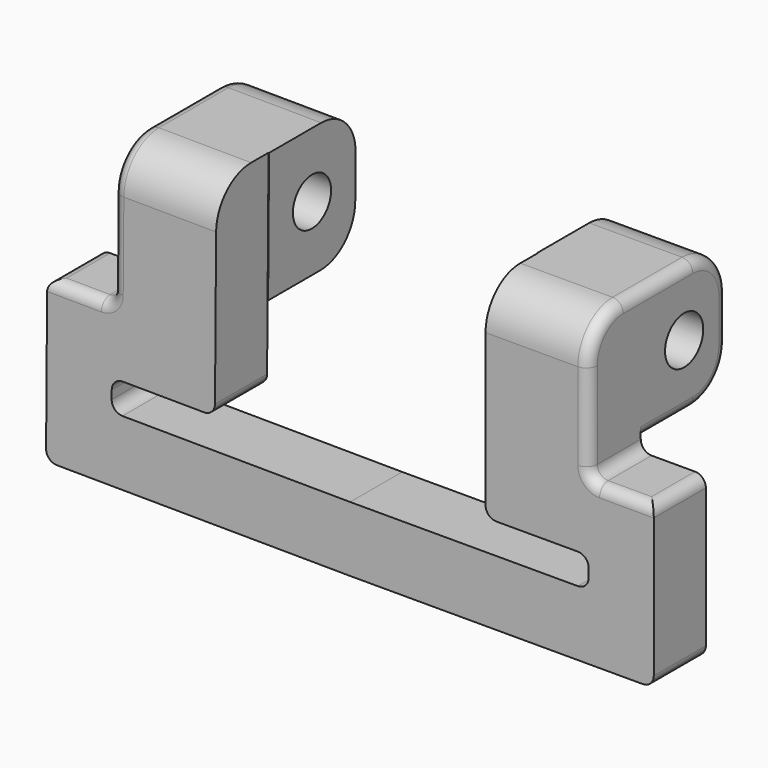
from build123d import *

# Parameters (mm, degrees)
F1_DEPTH = 3
F2_W     = 5
F2_H     = 6
F3_DEPTH = 4.775
F4_D     = 2.2
F5_R     = 2
F6_R     = 0.5


# Not quite as in the source:
# - a feature names something its author has since deleted; it is built from what else it names


with BuildPart() as f1:
    # F0 (on Front) → F1 (new body)
    with BuildSketch(Plane.XZ):
        Polygon((0.0109257422, 3), (0, 0), (14, 0), (14, 7.4), (11, 7.4), (11, 13.9), (6.25, 13.9), (6.25, 4.4), (11, 4.4), (11, 3), align=None)
    extrude(amount=F1_DEPTH)

    # F2 (on face) → F3 (join)
    with BuildSketch(Plane.YZ.offset(11)):
        with Locations((2.5, 10.9)):
            Rectangle(F2_W, F2_H)
    extrude(amount=-F3_DEPTH)

    # F4 (through all)
    with Locations(Plane.YZ.offset(11)):
        with Locations((2.5, 10.9)):
            Hole(F4_D / 2)

    # F5
    f5_edges = [f1.edges().sort_by_distance(p)[0] for p in [
        (8.6125, 5, 13.9),
        (8.6125, 5, 7.9),
        (8.625, -3, 13.9),
    ]]
    fillet(f5_edges, radius=F5_R)

    # F6 (call 1 of 5: OpenCascade refuses the feature's edges together)
    f6_edges = [f1.edges().sort_by_distance(p)[0] for p in [
        (14, -1.5, 7.4),
        (11, -1.5, 7.4),
        (11, 1, 13.9),
        (11, -3, 9.65),
        (12.5, -3, 7.4),
        (11, -2.414214, 13.314214),
        (11, 4.414214, 13.314214),
        (11, 1.5, 7.9),
        (11, 5, 10.9),
        (11, 4.414214, 8.485786),
    ]]
    fillet(f6_edges, radius=F6_R)

    # F6#2 (call 2 of 5)
    f6_2_edges = [f1.edges().sort_by_distance(p)[0] for p in [
        (6.25, -1.5, 4.4),
    ]]
    fillet(f6_2_edges, radius=F6_R)

    # F6#3 (call 3 of 5)
    f6_3_edges = [f1.edges().sort_by_distance(p)[0] for p in [
        (14, -1.5, 0),
    ]]
    fillet(f6_3_edges, radius=F6_R)

    # F6#4 (call 4 of 5)
    f6_4_edges = [f1.edges().sort_by_distance(p)[0] for p in [
        (11, -1.5, 4.4),
    ]]
    fillet(f6_4_edges, radius=F6_R)

    # F6#5 (call 5 of 5)
    f6_5_edges = [f1.edges().sort_by_distance(p)[0] for p in [
        (11, -1.5, 3),
    ]]
    fillet(f6_5_edges, radius=F6_R)

    # F7: F1 across face


with BuildPart() as f1_1:
    add(f1.part)
    add(f1.part.mirror(Plane(origin=(0.0054628711, -1.5, 1.5), x_dir=(0, -1, 0), z_dir=(-0.9999933683, 0, 0.0036418899))))


solid = f1_1.part
